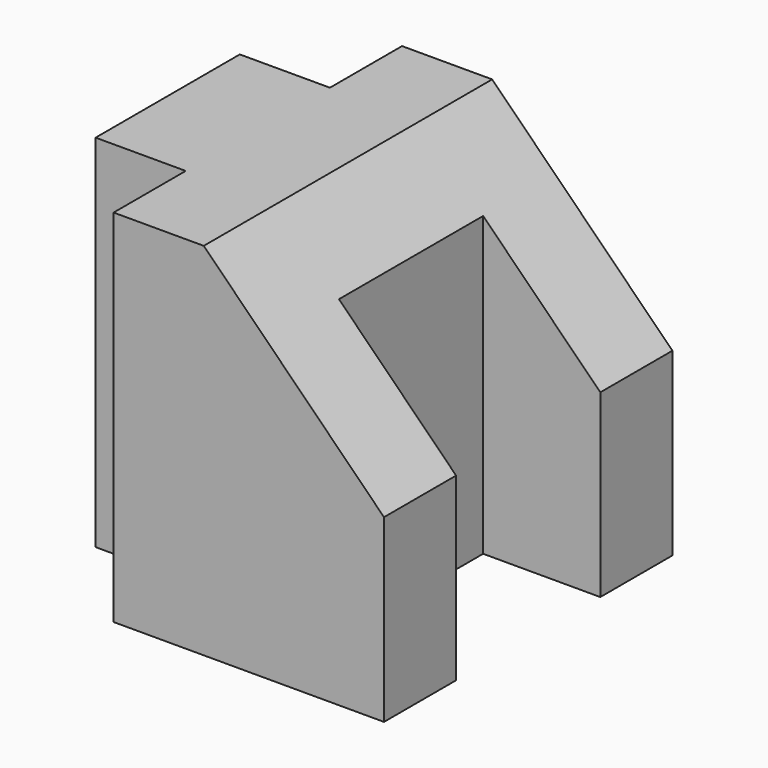
from build123d import *

# Parameters (mm, degrees)
F0_W     = 12.7
F0_H     = 50.8
F1_DEPTH = 25.4
F2_W     = 12.7
F2_H     = 12.7
F2_W_2   = 16.51
F2_H_2   = 25.4
F3_DEPTH = 50.801


# Not quite as in the source:
# - a feature names something its author has since deleted; it is built from what else it names


with BuildPart() as f1:
    # F0 (on Front) → F1 (new body, symmetric)
    with BuildSketch(Plane.XZ):
        with Locations((6.35, 25.4)):
            Rectangle(F0_W, F0_H)
        Polygon((12.7, 50.8), (12.7, 0), (25.4, 0), (50.8, 0), (50.8, 25.4), (25.4, 50.8), align=None)
    extrude(amount=F1_DEPTH, both=True)

    # F2 (on face) → F3 (cut, through all)
    with BuildSketch(Plane.XY.offset(50.8)):
        with Locations((6.35, -19.05)):
            Rectangle(F2_W, F2_H)
        with Locations((6.35, 19.05)):
            Rectangle(F2_W, F2_H)
        with Locations((42.545, 0)):
            Rectangle(F2_W_2, F2_H_2)
    extrude(amount=-F3_DEPTH, mode=Mode.SUBTRACT)


solid = f1.part
